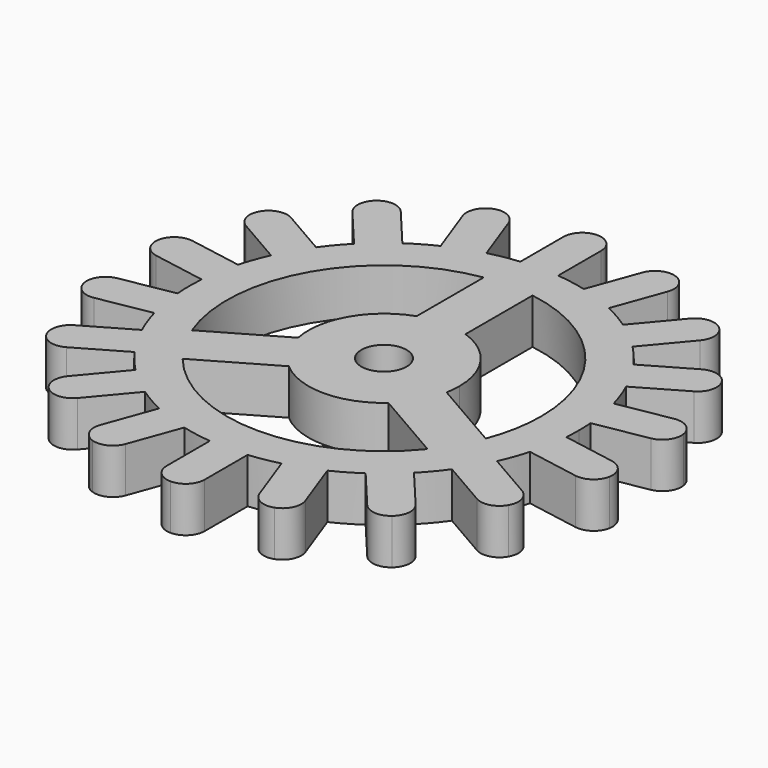
from build123d import *

# Parameters (mm, degrees)
F0_R     = 7.5
F0_R_2   = 3
F1_DEPTH = 6
F2_DEPTH = 2


with BuildPart() as f1:
    # F0 (on Top) → F1 (new body)
    with BuildSketch(Plane.XY):
        with BuildLine():
            Line((2.5, 0), (-2.5, 0))
            ThreePointArc((-2.5, 0), (-4.4830879458, -0.2708903524), (-6.4392310121, -0.6945927107))
            Line((-6.4392310121, -0.6945927107), (-11.137694116, -2.4046934273))
            ThreePointArc((-11.137694116, -2.4046934273), (-12.9085372679, -3.3375031159), (-14.6017957311, -4.4046934273))
            Line((-14.6017957311, -4.4046934273), (-18.4320179467, -7.6186314757))
            ThreePointArc((-18.4320179467, -7.6186314757), (-19.7770264858, -9.1008498853), (-21.0031683855, -10.6828092482))
            Line((-21.0031683855, -10.6828092482), (-23.5031683855, -15.0129362671))
            ThreePointArc((-23.5031683855, -15.0129362671), (-24.2601144316, -16.8657859823), (-24.8712489588, -18.7717067503))
            Line((-24.8712489588, -18.7717067503), (-25.7394898471, -23.6957455153))
            ThreePointArc((-25.7394898471, -23.6957455153), (-25.8170745358, -25.6957455153), (-25.7394898471, -27.6957455153))
            Line((-25.7394898471, -27.6957455153), (-24.8712489588, -32.6197842804))
            ThreePointArc((-24.8712489588, -32.6197842804), (-24.2601144316, -34.5257050483), (-23.5031683855, -36.3785547636))
            Line((-23.5031683855, -36.3785547636), (-21.0031683855, -40.7086817825))
            ThreePointArc((-21.0031683855, -40.7086817825), (-19.7770264858, -42.2906411453), (-18.4320179467, -43.772859555))
            Line((-18.4320179467, -43.772859555), (-14.6017957311, -46.9867976034))
            ThreePointArc((-14.6017957311, -46.9867976034), (-12.9085372679, -48.0539879148), (-11.137694116, -48.9867976034))
            Line((-11.137694116, -48.9867976034), (-6.4392310121, -50.69689832))
            ThreePointArc((-6.4392310121, -50.69689832), (-4.4830879458, -51.1206006783), (-2.5, -51.3914910307))
            Line((-2.5, -51.3914910307), (2.5, -51.3914910307))
            ThreePointArc((2.5, -51.3914910307), (4.4830879458, -51.1206006783), (6.4392310121, -50.69689832))
            Line((6.4392310121, -50.69689832), (11.137694116, -48.9867976034))
            ThreePointArc((11.137694116, -48.9867976034), (12.9085372679, -48.0539879148), (14.6017957311, -46.9867976034))
            Line((14.6017957311, -46.9867976034), (18.4320179467, -43.772859555))
            ThreePointArc((18.4320179467, -43.772859555), (19.7770264858, -42.2906411453), (21.0031683855, -40.7086817825))
            Line((21.0031683855, -40.7086817825), (23.5031683855, -36.3785547636))
            ThreePointArc((23.5031683855, -36.3785547636), (24.2601144316, -34.5257050483), (24.8712489588, -32.6197842804))
            Line((24.8712489588, -32.6197842804), (25.7394898471, -27.6957455153))
            ThreePointArc((25.7394898471, -27.6957455153), (25.7976710721, -26.6964976555), (25.8170745358, -25.6957455153))
            ThreePointArc((25.8170745358, -25.6957455153), (25.7976710721, -24.6949933752), (25.7394898471, -23.6957455153))
            Line((25.7394898471, -23.6957455153), (24.8712489588, -18.7717067503))
            ThreePointArc((24.8712489588, -18.7717067503), (24.2601144316, -16.8657859823), (23.5031683855, -15.0129362671))
            Line((23.5031683855, -15.0129362671), (21.0031683855, -10.6828092482))
            ThreePointArc((21.0031683855, -10.6828092482), (19.7770264858, -9.1008498853), (18.4320179467, -7.6186314757))
            Line((18.4320179467, -7.6186314757), (14.6017957311, -4.4046934273))
            ThreePointArc((14.6017957311, -4.4046934273), (12.9085372679, -3.3375031159), (11.137694116, -2.4046934273))
            Line((11.137694116, -2.4046934273), (6.4392310121, -0.6945927107))
            ThreePointArc((6.4392310121, -0.6945927107), (4.4830879458, -0.2708903524), (2.5, 0))
        make_face()
        with BuildLine():
            ThreePointArc((3.2092747543, -5.1275383066), (15.8138911087, -12.1579672548), (20.8170745358, -25.6957455153))
            ThreePointArc((20.8170745358, -25.6957455153), (20.4679370808, -29.4923418708), (19.4322359639, -33.161587576))
            ThreePointArc((19.4322359639, -33.161587576), (18.0385412737, -36.0862036837), (16.2079525759, -38.7591625847))
            ThreePointArc((16.2079525759, -38.7591625847), (0.0208699061, -46.5128095898), (-16.1817268671, -38.791634482))
            ThreePointArc((-16.1817268671, -38.791634482), (-18.0176713676, -36.1223514214), (-19.4172273302, -33.2005356548))
            ThreePointArc((-19.4172273302, -33.2005356548), (-18.0385412737, -15.305287347), (-3.2505090967, -5.1340144879))
            ThreePointArc((-3.2505090967, -5.1340144879), (-0.0208699061, -4.8786814409), (3.2092747543, -5.1275383066))
        make_face(mode=Mode.SUBTRACT)
        with BuildLine():
            ThreePointArc((10, -25.6957455153), (8.1268920118, -19.8687714954), (3.2092747543, -16.2247077923))
            ThreePointArc((3.2092747543, -16.2247077923), (-0.0217847835, -15.6957692442), (-3.2505090967, -16.238780325))
            ThreePointArc((-3.2505090967, -16.238780325), (-8.6711258798, -20.7146235557), (-9.8067966455, -27.6519509119))
            ThreePointArc((-9.8067966455, -27.6519509119), (-8.6493410963, -30.7145998269), (-6.5647175492, -33.2392515635))
            ThreePointArc((-6.5647175492, -33.2392515635), (0.0217847835, -35.6957217865), (6.5975218912, -33.2105778418))
            ThreePointArc((6.5975218912, -33.2105778418), (8.6711258798, -30.676867475), (9.8152266459, -27.6092046575))
            ThreePointArc((9.8152266459, -27.6092046575), (9.9536994746, -26.6569253998), (10, -25.6957455153))
        make_face()
        with Locations((0, -25.6957455153)):
            Circle(F0_R, mode=Mode.SUBTRACT)
        with Locations((0, -25.6957455153)):
            Circle(F0_R)
        with Locations((0, -25.6957455153)):
            Circle(F0_R_2, mode=Mode.SUBTRACT)
        with BuildLine():
            Line((-9.8067966455, -27.6519509119), (-19.4172273302, -33.2005356548))
            ThreePointArc((-19.4172273302, -33.2005356548), (-18.0176713676, -36.1223514214), (-16.1817268671, -38.791634482))
            Line((-16.1817268671, -38.791634482), (-6.5647175492, -33.2392515635))
            ThreePointArc((-6.5647175492, -33.2392515635), (-8.6493410963, -30.7145998269), (-9.8067966455, -27.6519509119))
        make_face()
        with BuildLine():
            Line((3.2092747543, -16.2247077923), (3.2092747543, -5.1275383066))
            ThreePointArc((3.2092747543, -5.1275383066), (-0.0208699061, -4.8786814409), (-3.2505090967, -5.1340144879))
            Line((-3.2505090967, -5.1340144879), (-3.2505090967, -16.238780325))
            ThreePointArc((-3.2505090967, -16.238780325), (-0.0217847835, -15.6957692442), (3.2092747543, -16.2247077923))
        make_face()
        with BuildLine():
            ThreePointArc((16.2079525759, -38.7591625847), (18.0385412737, -36.0862036837), (19.4322359639, -33.161587576))
            Line((19.4322359639, -33.161587576), (9.8152266459, -27.6092046575))
            ThreePointArc((9.8152266459, -27.6092046575), (8.6711258798, -30.676867475), (6.5975218912, -33.2105778418))
            Line((6.5975218912, -33.2105778418), (16.2079525759, -38.7591625847))
        make_face()
        with BuildLine():
            Line((31.8727341228, -17.5371560108), (24.8712489588, -18.7717067503))
            ThreePointArc((24.8712489588, -18.7717067503), (25.424855163, -21.2126575695), (25.7394898471, -23.6957455153))
            Line((25.7394898471, -23.6957455153), (32.7409750112, -22.4611947759))
            ThreePointArc((32.7409750112, -22.4611947759), (34.3547346777, -21.4331164842), (34.7688739495, -19.5650549492))
            ThreePointArc((34.7688739495, -19.5650549492), (33.7407956579, -17.9512952826), (31.8727341228, -17.5371560108))
        make_face()
        with BuildLine():
            Line((23.0019128314, -49.2190482015), (18.4320179467, -43.772859555))
            ThreePointArc((18.4320179467, -43.772859555), (16.59489563, -45.4727720011), (14.6017957311, -46.9867976034))
            Line((14.6017957311, -46.9867976034), (19.1716906158, -52.43298625))
            ThreePointArc((19.1716906158, -52.43298625), (20.8689123667, -53.316503971), (22.6937707478, -52.7411283335))
            ThreePointArc((22.6937707478, -52.7411283335), (23.5772884688, -51.0439065826), (23.0019128314, -49.2190482015))
        make_face()
        with BuildLine():
            Line((13.5692843954, -55.6675369894), (11.137694116, -48.9867976034))
            ThreePointArc((11.137694116, -48.9867976034), (8.829959533, -49.955859947), (6.4392310121, -50.69689832))
            Line((6.4392310121, -50.69689832), (8.8708212915, -57.377637706))
            ThreePointArc((8.8708212915, -57.377637706), (10.1635071891, -58.7883568153), (12.0751032017, -58.8718188997))
            ThreePointArc((12.0751032017, -58.8718188997), (13.485822311, -57.5791330021), (13.5692843954, -55.6675369894))
        make_face()
        with BuildLine():
            ThreePointArc((2.5, -51.3914910307), (0, -51.5128200512), (-2.5, -51.3914910307))
            Line((-2.5, -51.3914910307), (-2.5, -58.500985389))
            ThreePointArc((-2.5, -58.500985389), (-1.767766953, -60.268752342), (0, -61.000985389))
            ThreePointArc((0, -61.000985389), (1.767766953, -60.268752342), (2.5, -58.500985389))
            Line((2.5, -58.500985389), (2.5, -51.3914910307))
        make_face()
        with BuildLine():
            ThreePointArc((-6.4392310121, -50.69689832), (-8.829959533, -49.955859947), (-11.137694116, -48.9867976034))
            Line((-11.137694116, -48.9867976034), (-13.5692843954, -55.6675369894))
            ThreePointArc((-13.5692843954, -55.6675369894), (-13.485822311, -57.5791330021), (-12.0751032017, -58.8718188997))
            ThreePointArc((-12.0751032017, -58.8718188997), (-10.1635071891, -58.7883568153), (-8.8708212915, -57.377637706))
            Line((-8.8708212915, -57.377637706), (-6.4392310121, -50.69689832))
        make_face()
        with BuildLine():
            ThreePointArc((-14.6017957311, -46.9867976034), (-16.59489563, -45.4727720011), (-18.4320179467, -43.772859555))
            Line((-18.4320179467, -43.772859555), (-23.0019128314, -49.2190482015))
            ThreePointArc((-23.0019128314, -49.2190482015), (-23.5772884688, -51.0439065826), (-22.6937707478, -52.7411283335))
            ThreePointArc((-22.6937707478, -52.7411283335), (-20.8689123667, -53.316503971), (-19.1716906158, -52.43298625))
            Line((-19.1716906158, -52.43298625), (-14.6017957311, -46.9867976034))
        make_face()
        with BuildLine():
            ThreePointArc((-21.0031683855, -40.7086817825), (-22.3582423994, -38.6042827833), (-23.5031683855, -36.3785547636))
            Line((-23.5031683855, -36.3785547636), (-29.6601711078, -39.9333019427))
            ThreePointArc((-29.6601711078, -39.9333019427), (-30.8249856736, -41.4513178394), (-30.5752346173, -43.3483654522))
            ThreePointArc((-30.5752346173, -43.3483654522), (-29.0572187206, -44.5131800179), (-27.1601711078, -44.2634289616))
            Line((-27.1601711078, -44.2634289616), (-21.0031683855, -40.7086817825))
        make_face()
        with BuildLine():
            ThreePointArc((-24.8712489588, -32.6197842804), (-25.424855163, -30.1788334612), (-25.7394898471, -27.6957455153))
            Line((-25.7394898471, -27.6957455153), (-32.7409750112, -28.9302962548))
            ThreePointArc((-32.7409750112, -28.9302962548), (-34.3547346777, -29.9583745465), (-34.7688739495, -31.8264360815))
            ThreePointArc((-34.7688739495, -31.8264360815), (-33.7407956579, -33.4401957481), (-31.8727341228, -33.8543350199))
            Line((-31.8727341228, -33.8543350199), (-24.8712489588, -32.6197842804))
        make_face()
        with BuildLine():
            ThreePointArc((-25.7394898471, -23.6957455153), (-25.424855163, -21.2126575695), (-24.8712489588, -18.7717067503))
            Line((-24.8712489588, -18.7717067503), (-31.8727341228, -17.5371560108))
            ThreePointArc((-31.8727341228, -17.5371560108), (-33.7407956579, -17.9512952826), (-34.7688739495, -19.5650549492))
            ThreePointArc((-34.7688739495, -19.5650549492), (-34.3547346777, -21.4331164842), (-32.7409750112, -22.4611947759))
            Line((-32.7409750112, -22.4611947759), (-25.7394898471, -23.6957455153))
        make_face()
        with BuildLine():
            ThreePointArc((-23.5031683855, -15.0129362671), (-22.3582423994, -12.7872082474), (-21.0031683855, -10.6828092482))
            Line((-21.0031683855, -10.6828092482), (-27.1601711078, -7.1280620691))
            ThreePointArc((-27.1601711078, -7.1280620691), (-29.0572187206, -6.8783110128), (-30.5752346173, -8.0431255785))
            ThreePointArc((-30.5752346173, -8.0431255785), (-30.8249856736, -9.9401731913), (-29.6601711078, -11.458189088))
            Line((-29.6601711078, -11.458189088), (-23.5031683855, -15.0129362671))
        make_face()
        with BuildLine():
            ThreePointArc((-18.4320179467, -7.6186314757), (-16.59489563, -5.9187190296), (-14.6017957311, -4.4046934273))
            Line((-14.6017957311, -4.4046934273), (-19.1716906158, 1.0414952193))
            ThreePointArc((-19.1716906158, 1.0414952193), (-20.8689123667, 1.9250129403), (-22.6937707478, 1.3496373028))
            ThreePointArc((-22.6937707478, 1.3496373029), (-23.5772884688, -0.3475844481), (-23.0019128314, -2.1724428292))
            Line((-23.0019128314, -2.1724428292), (-18.4320179467, -7.6186314757))
        make_face()
        with BuildLine():
            ThreePointArc((-11.137694116, -2.4046934273), (-8.829959533, -1.4356310837), (-6.4392310121, -0.6945927107))
            Line((-6.4392310121, -0.6945927107), (-8.8708212915, 5.9861466754))
            ThreePointArc((-8.8708212915, 5.9861466754), (-10.1635071891, 7.3968657846), (-12.0751032017, 7.480327869))
            ThreePointArc((-12.0751032017, 7.480327869), (-13.485822311, 6.1876419714), (-13.5692843954, 4.2760459587))
            Line((-13.5692843954, 4.2760459587), (-11.137694116, -2.4046934273))
        make_face()
        with BuildLine():
            Line((-2.5, 7.1094943583), (-2.5, 0))
            ThreePointArc((-2.5, 0), (0, 0.1213290205), (2.5, 0))
            Line((2.5, 0), (2.5, 7.1094943583))
            ThreePointArc((2.5, 7.1094943583), (1.767766953, 8.8772613113), (0, 9.6094943583))
            ThreePointArc((0, 9.6094943583), (-1.767766953, 8.8772613113), (-2.5, 7.1094943583))
        make_face()
        with BuildLine():
            Line((19.1716906158, 1.0414952193), (14.6017957311, -4.4046934273))
            ThreePointArc((14.6017957311, -4.4046934273), (16.59489563, -5.9187190296), (18.4320179467, -7.6186314757))
            Line((18.4320179467, -7.6186314757), (23.0019128314, -2.1724428292))
            ThreePointArc((23.0019128314, -2.1724428292), (23.5772884688, -0.3475844481), (22.6937707478, 1.3496373029))
            ThreePointArc((22.6937707478, 1.3496373028), (20.8689123667, 1.9250129403), (19.1716906158, 1.0414952193))
        make_face()
        with BuildLine():
            Line((27.1601711078, -7.1280620691), (21.0031683855, -10.6828092482))
            ThreePointArc((21.0031683855, -10.6828092482), (22.3582423994, -12.7872082474), (23.5031683855, -15.0129362671))
            Line((23.5031683855, -15.0129362671), (29.6601711078, -11.458189088))
            ThreePointArc((29.6601711078, -11.458189088), (30.8249856736, -9.9401731913), (30.5752346173, -8.0431255785))
            ThreePointArc((30.5752346173, -8.0431255785), (29.0572187206, -6.8783110128), (27.1601711078, -7.1280620691))
        make_face()
        with BuildLine():
            Line((8.8708212915, 5.9861466754), (6.4392310121, -0.6945927107))
            ThreePointArc((6.4392310121, -0.6945927107), (8.829959533, -1.4356310837), (11.137694116, -2.4046934273))
            Line((11.137694116, -2.4046934273), (13.5692843954, 4.2760459587))
            ThreePointArc((13.5692843954, 4.2760459587), (13.485822311, 6.1876419714), (12.0751032017, 7.480327869))
            ThreePointArc((12.0751032017, 7.480327869), (10.1635071891, 7.3968657846), (8.8708212915, 5.9861466754))
        make_face()
        with BuildLine():
            Line((32.7409750112, -28.9302962548), (25.7394898471, -27.6957455153))
            ThreePointArc((25.7394898471, -27.6957455153), (25.424855163, -30.1788334612), (24.8712489588, -32.6197842804))
            Line((24.8712489588, -32.6197842804), (31.8727341228, -33.8543350199))
            ThreePointArc((31.8727341228, -33.8543350199), (33.7407956579, -33.4401957481), (34.7688739495, -31.8264360815))
            ThreePointArc((34.7688739495, -31.8264360815), (34.3547346777, -29.9583745465), (32.7409750112, -28.9302962548))
        make_face()
        with BuildLine():
            Line((29.6601711078, -39.9333019427), (23.5031683855, -36.3785547636))
            ThreePointArc((23.5031683855, -36.3785547636), (22.3582423994, -38.6042827833), (21.0031683855, -40.7086817825))
            Line((21.0031683855, -40.7086817825), (27.1601711078, -44.2634289616))
            ThreePointArc((27.1601711078, -44.2634289616), (29.0572187206, -44.5131800179), (30.5752346173, -43.3483654522))
            ThreePointArc((30.5752346173, -43.3483654522), (30.8249856736, -41.4513178394), (29.6601711078, -39.9333019427))
        make_face()
        with BuildLine():
            Line((-24.8712489588, -32.6197842804), (-25.7394898471, -27.6957455153))
            ThreePointArc((-25.7394898471, -27.6957455153), (-25.424855163, -30.1788334612), (-24.8712489588, -32.6197842804))
        make_face()
        with BuildLine():
            Line((-23.5031683855, -15.0129362671), (-21.0031683855, -10.6828092482))
            ThreePointArc((-21.0031683855, -10.6828092482), (-22.3582423994, -12.7872082474), (-23.5031683855, -15.0129362671))
        make_face()
        with BuildLine():
            Line((-6.4392310121, -50.69689832), (-11.137694116, -48.9867976034))
            ThreePointArc((-11.137694116, -48.9867976034), (-8.829959533, -49.955859947), (-6.4392310121, -50.69689832))
        make_face()
        with BuildLine():
            Line((-18.4320179467, -7.6186314757), (-14.6017957311, -4.4046934273))
            ThreePointArc((-14.6017957311, -4.4046934273), (-16.59489563, -5.9187190296), (-18.4320179467, -7.6186314757))
        make_face()
        with BuildLine():
            ThreePointArc((24.8712489588, -32.6197842804), (25.424855163, -30.1788334612), (25.7394898471, -27.6957455153))
            Line((25.7394898471, -27.6957455153), (24.8712489588, -32.6197842804))
        make_face()
        with BuildLine():
            Line((-11.137694116, -2.4046934273), (-6.4392310121, -0.6945927107))
            ThreePointArc((-6.4392310121, -0.6945927107), (-8.829959533, -1.4356310837), (-11.137694116, -2.4046934273))
        make_face()
        with BuildLine():
            ThreePointArc((21.0031683855, -40.7086817825), (22.3582423994, -38.6042827833), (23.5031683855, -36.3785547636))
            Line((23.5031683855, -36.3785547636), (21.0031683855, -40.7086817825))
        make_face()
        with BuildLine():
            ThreePointArc((2.5, 0), (0, 0.1213290205), (-2.5, 0))
            Line((-2.5, 0), (2.5, 0))
        make_face()
        with BuildLine():
            ThreePointArc((11.137694116, -2.4046934273), (8.829959533, -1.4356310837), (6.4392310121, -0.6945927107))
            Line((6.4392310121, -0.6945927107), (11.137694116, -2.4046934273))
        make_face()
        with BuildLine():
            ThreePointArc((18.4320179467, -7.6186314757), (16.59489563, -5.9187190296), (14.6017957311, -4.4046934273))
            Line((14.6017957311, -4.4046934273), (18.4320179467, -7.6186314757))
        make_face()
        with BuildLine():
            ThreePointArc((23.5031683855, -15.0129362671), (22.3582423994, -12.7872082474), (21.0031683855, -10.6828092482))
            Line((21.0031683855, -10.6828092482), (23.5031683855, -15.0129362671))
        make_face()
        with BuildLine():
            Line((-21.0031683855, -40.7086817825), (-23.5031683855, -36.3785547636))
            ThreePointArc((-23.5031683855, -36.3785547636), (-22.3582423994, -38.6042827833), (-21.0031683855, -40.7086817825))
        make_face()
        with BuildLine():
            Line((2.5, -51.3914910307), (-2.5, -51.3914910307))
            ThreePointArc((-2.5, -51.3914910307), (0, -51.5128200512), (2.5, -51.3914910307))
        make_face()
        with BuildLine():
            ThreePointArc((25.7394898471, -23.6957455153), (25.424855163, -21.2126575695), (24.8712489588, -18.7717067503))
            Line((24.8712489588, -18.7717067503), (25.7394898471, -23.6957455153))
        make_face()
        with BuildLine():
            ThreePointArc((6.4392310121, -50.69689832), (8.829959533, -49.955859947), (11.137694116, -48.9867976034))
            Line((11.137694116, -48.9867976034), (6.4392310121, -50.69689832))
        make_face()
        with BuildLine():
            Line((-14.6017957311, -46.9867976034), (-18.4320179467, -43.772859555))
            ThreePointArc((-18.4320179467, -43.772859555), (-16.59489563, -45.4727720011), (-14.6017957311, -46.9867976034))
        make_face()
        with BuildLine():
            Line((-25.7394898471, -23.6957455153), (-24.8712489588, -18.7717067503))
            ThreePointArc((-24.8712489588, -18.7717067503), (-25.424855163, -21.2126575695), (-25.7394898471, -23.6957455153))
        make_face()
        with BuildLine():
            ThreePointArc((14.6017957311, -46.9867976034), (16.59489563, -45.4727720011), (18.4320179467, -43.772859555))
            Line((18.4320179467, -43.772859555), (14.6017957311, -46.9867976034))
        make_face()
    extrude(amount=F1_DEPTH)

    # F0 (on Top) → F2 (join)
    with BuildSketch(Plane.XY):
        with Locations((0, -25.6957455153)):
            Circle(F0_R)
        with Locations((0, -25.6957455153)):
            Circle(F0_R_2, mode=Mode.SUBTRACT)
    extrude(amount=-F2_DEPTH)


solid = f1.part
